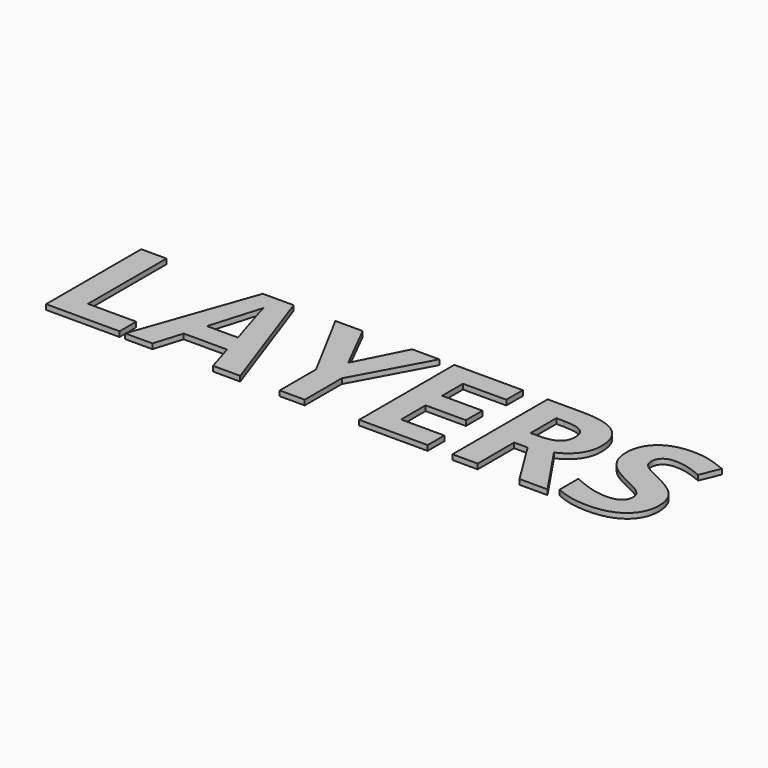
from build123d import *

# Parameters (mm, degrees)
F0_TEXT_SIZE = 41.4658617465
F1_DEPTH     = 1.27


# Not quite as in the source:
# - Text() gives the source's letters only with a copy of the font that has no kerning and outlines rounded to 1/6400 em; it was checked with that copy


with BuildPart() as f1:
    # F0 (on Top) → F1 (new body)
    with BuildSketch(Plane.XY):
        with Locations((-45.6686749712, -11.3855419092)):
            Text('LAYERS', F0_TEXT_SIZE, font='Open Sans', font_style=FontStyle.BOLD, text_align=(TextAlign.LEFT, TextAlign.BOTTOM))
    extrude(amount=F1_DEPTH)


solid = f1.part
